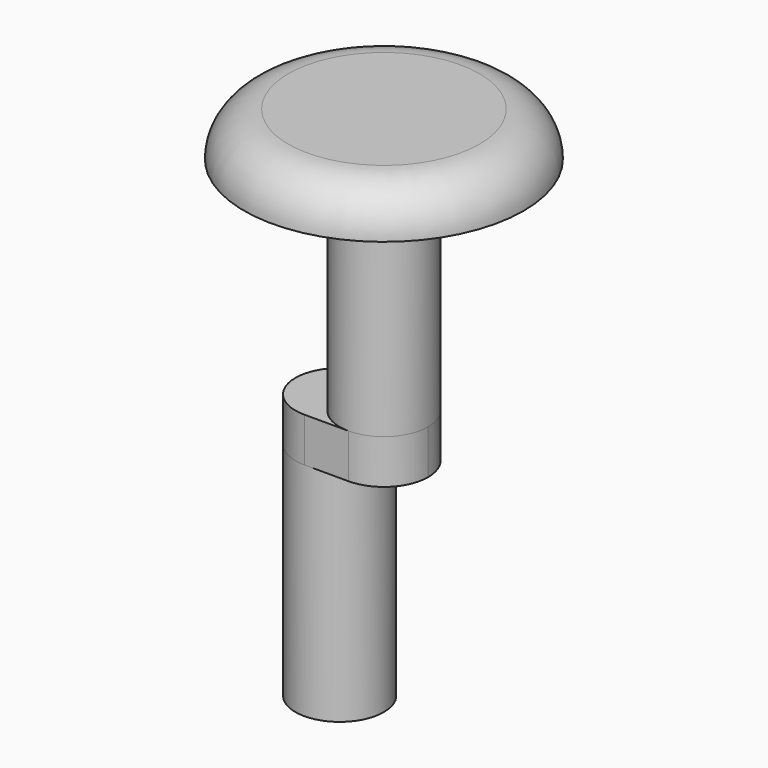
from build123d import *

# Parameters (mm, degrees)
F0_R     = 5
F1_DEPTH = 25
F2_W     = 15
F2_H     = 10
F3_DEPTH = 5
F4_R     = 5
F5_DEPTH = 25
F6_R     = 4.9999
F7_R     = 15.7954316655
F8_DEPTH = 5
F9_R     = 4.99999


# Not quite as in the source:
# - a fillet or chamfer is up to 0.001 mm smaller than in the source, because OpenCascade refuses the exact size


with BuildPart() as f1:
    # F0 (on Top) → F1 (new body)
    with BuildSketch(Plane.XY):
        Circle(F0_R)
    extrude(amount=F1_DEPTH)

    # F2 (on face) → F3 (join)
    with BuildSketch(Plane.XY.offset(25)):
        with Locations((2.5, 0)):
            Rectangle(F2_W, F2_H)
    extrude(amount=F3_DEPTH)

    # F4 (on face) → F5 (join)
    with BuildSketch(Plane.XY.offset(30)):
        with Locations((5, 0)):
            Circle(F4_R)
    extrude(amount=F5_DEPTH)

    # F6 (radius 5 in the source; OpenCascade refuses exactly that, so slightly less here)
    f6_edges = [f1.edges().sort_by_distance(p)[0] for p in [
        (10, -5, 27.5),
        (10, 5, 27.5),
        (-5, 5, 27.5),
        (-5, -5, 27.5),
    ]]
    fillet(f6_edges, radius=F6_R)

    # F7 (on face) → F8 (join)
    with BuildSketch(Plane.XY.offset(55)):
        with Locations((5, 0)):
            Circle(F7_R)
    extrude(amount=F8_DEPTH)

    # F9 (radius 5 in the source; OpenCascade refuses exactly that, so slightly less here)
    f9_edges = [f1.edges().sort_by_distance(p)[0] for p in [
        (-10.795432, 0, 60),
    ]]
    fillet(f9_edges, radius=F9_R)


solid = f1.part
